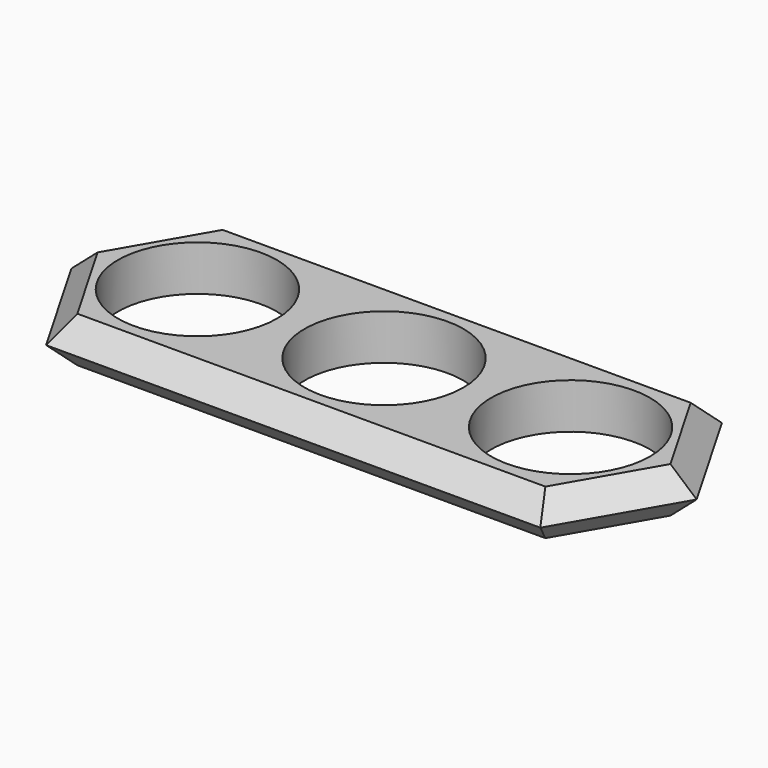
from build123d import *

# Parameters (mm, degrees)
F1_DEPTH = 6.35
F3_SIZE  = 3.17499
F4_SIZE  = 3.17499
F2_R     = 11.1125
F5_DEPTH = 25.4
F6_R     = 11.1125
F7_DEPTH = 25.4


# Not quite as in the source:
# - a fillet or chamfer is up to 0.001 mm smaller than in the source, because OpenCascade refuses the exact size


with BuildPart() as f1:
    # F0 (on Top) → F1 (new body)
    with BuildSketch(Plane.XY):
        Polygon((25.4, -15.875), (25.4, 15.875), (16.2345644766, 15.875), (7.0691289532, 0), (16.2345644766, -15.875), align=None)
        Polygon((34.5654355234, 15.875), (25.4, 15.875), (25.4, -15.875), (34.5654355234, -15.875), (43.7308710468, 0), align=None)
        Polygon((7.0691289532, 0), (16.2345644766, 15.875), (-16.2345644766, 15.875), (-7.0691289532, 0), (-16.2345644766, -15.875), (16.2345644766, -15.875), align=None)
        Polygon((-7.0691289532, 0), (-16.2345644766, 15.875), (-25.4, 15.875), (-25.4, -15.875), (-16.2345644766, -15.875), align=None)
        Polygon((-25.4, -15.875), (-25.4, 15.875), (-34.5654355234, 15.875), (-43.7308710468, 0), (-34.5654355234, -15.875), align=None)
    extrude(amount=F1_DEPTH)

    # F3 (size 3.175 in the source; OpenCascade refuses exactly that, so slightly less here)
    f3_edges = [f1.edges().sort_by_distance(p)[0] for p in [
        (-39.148153, -7.9375, 0),
        (-39.148153, 7.9375, 6.35),
        (-39.148153, -7.9375, 6.35),
        (-39.148153, 7.9375, 0),
        (39.148153, -7.9375, 6.35),
        (39.148153, 7.9375, 6.35),
        (39.148153, 7.9375, 0),
        (39.148153, -7.9375, 0),
    ]]
    chamfer(f3_edges, length=F3_SIZE)

    # F4 (size 3.175 in the source; OpenCascade refuses exactly that, so slightly less here)
    f4_edges = [f1.edges().sort_by_distance(p)[0] for p in [
        (0, 15.875, 0),
        (0, 15.875, 6.35),
        (0, -15.875, 6.35),
        (0, -15.875, 0),
    ]]
    chamfer(f4_edges, length=F4_SIZE)

    # F2 (on Top) → F5 (cut)
    with BuildSketch(Plane.XY):
        Circle(F2_R)
    extrude(amount=F5_DEPTH, mode=Mode.SUBTRACT)

    # F6 (on Top) → F7 (cut)
    with BuildSketch(Plane.XY):
        with Locations((26.0964684711, 0)):
            Circle(F6_R)
        with Locations((-26.0964684711, 0)):
            Circle(F6_R)
    extrude(amount=F7_DEPTH, mode=Mode.SUBTRACT)


solid = f1.part
